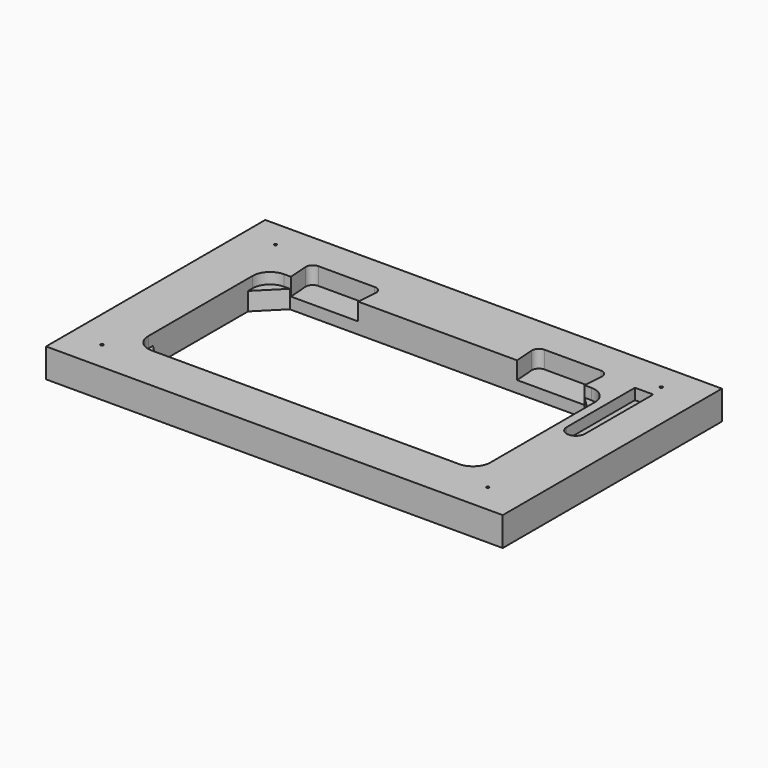
from build123d import *

# Parameters (mm, degrees)
F0_W     = 500
F0_H     = 300
F1_DEPTH = 31.75
F2_R     = 1.5
F3_DEPTH = 31.751
F5_DEPTH = 12
F8_DEPTH = 31.751
F9_DEPTH = 19.05


# Not quite as in the source:
# - a length typed as a fraction of an inch, garbled in the dataset ("3 / 203.2 mm" for 3/8 in), is restored


with BuildPart() as f1:
    # F0 (on Top) → F1 (new body)
    with BuildSketch(Plane.XY):
        Rectangle(F0_W, F0_H)
    extrude(amount=-F1_DEPTH)

    # F2 (on Top) → F3 (cut, through all)
    with BuildSketch(Plane.XY):
        with Locations((-214.6335691214, 119.7834908962)):
            Circle(F2_R)
        with Locations((-214.6335691214, -117.7065091038)):
            Circle(F2_R)
        with Locations((207.7684308786, 119.7834908962)):
            Circle(F2_R)
        with Locations((207.7684308786, -117.7065091038)):
            Circle(F2_R)
        with Locations((630.1704308786, 119.7834908962)):
            Circle(F2_R)
        with Locations((630.1704308786, -117.7065091038)):
            Circle(F2_R)
    extrude(amount=-F3_DEPTH, mode=Mode.SUBTRACT)

    # F4 (on Top) → F5 (cut)
    with BuildSketch(Plane.XY):
        with BuildLine():
            ThreePointArc((-193.759300375, -80.4257169581), (-188.1796845566, -93.8961011397), (-174.709300375, -99.4757169581))
            Line((-174.709300375, -99.4757169581), (161.840699625, -99.4757169581))
            ThreePointArc((161.840699625, -99.4757169581), (175.3110838066, -93.8961011397), (180.890699625, -80.4257169581))
            Line((180.890699625, -80.4257169581), (180.890699625, 62.4492830419))
            ThreePointArc((180.890699625, 62.4492830419), (175.3110838066, 75.9196672235), (161.840699625, 81.4992830419))
            Line((161.840699625, 81.4992830419), (-174.709300375, 81.4992830419))
            ThreePointArc((-174.709300375, 81.4992830419), (-188.1796845566, 75.9196672235), (-193.759300375, 62.4492830419))
            Line((-193.759300375, 62.4492830419), (-193.759300375, -80.4257169581))
        make_face()
        with BuildLine():
            Line((210.890699625, 104.8424765468), (190.890699625, 104.8424765468))
            Line((190.890699625, 104.8424765468), (190.890699625, 11.4992830419))
            ThreePointArc((190.890699625, 11.4992830419), (200.890699625, 1.4992830419), (210.890699625, 11.4992830419))
            Line((210.890699625, 11.4992830419), (210.890699625, 104.8424765468))
        make_face()
    extrude(amount=-F5_DEPTH, mode=Mode.SUBTRACT)

    # F7 (on face) → F8 (cut, through all)
    with BuildSketch(Plane.XY):
        with BuildLine():
            Line((-174.709300375, -93.1257169581), (140.1676505526, -93.1257169581))
            Line((140.1676505526, -93.1257169581), (163.0281784434, -99.438670281))
            ThreePointArc((163.0281784434, -99.438670281), (175.7245746513, -93.4695091312), (180.890699625, -80.4257169581))
            Line((180.890699625, -80.4257169581), (180.890699625, 56.0992830419))
            Line((180.890699625, 56.0992830419), (154.220699625, 81.4992830419))
            Line((154.220699625, 81.4992830419), (-168.359300375, 81.4992830419))
            Line((-168.359300375, 81.4992830419), (-187.409300375, 62.4492830419))
            Line((-187.409300375, 62.4492830419), (-193.759300375, 56.0992830419))
            Line((-193.759300375, 56.0992830419), (-193.759300375, -74.0757169581))
            Line((-193.759300375, -74.0757169581), (-174.709300375, -93.1257169581))
        make_face()
    extrude(amount=-F8_DEPTH, mode=Mode.SUBTRACT)

    # F6 (on Top) → F9 (cut)
    with BuildSketch(Plane.XY):
        with BuildLine():
            ThreePointArc((-161.120300375, 111.4992830419), (-166.7055905698, 109.0628082362), (-168.7191172889, 103.3114965432))
            Line((-168.7191172889, 103.3114965432), (-167.089300375, 81.4992830419))
            Line((-167.089300375, 81.4992830419), (-93.429300375, 81.4992830419))
            Line((-93.429300375, 81.4992830419), (-91.799483461, 103.3114965432))
            ThreePointArc((-91.799483461, 103.3114965432), (-93.8130101802, 109.0628082362), (-99.398300375, 111.4992830419))
            Line((-99.398300375, 111.4992830419), (-161.120300375, 111.4992830419))
        make_face()
        with BuildLine():
            Line((148.251699625, 111.4992830419), (86.529699625, 111.4992830419))
            ThreePointArc((86.529699625, 111.4992830419), (80.9444094302, 109.0628082362), (78.9308827111, 103.3114965432))
            Line((78.9308827111, 103.3114965432), (80.560699625, 81.4992830419))
            Line((80.560699625, 81.4992830419), (154.220699625, 81.4992830419))
            Line((154.220699625, 81.4992830419), (155.850516539, 103.3114965432))
            ThreePointArc((155.850516539, 103.3114965432), (153.8369898198, 109.0628082362), (148.251699625, 111.4992830419))
        make_face()
    extrude(amount=-F9_DEPTH, mode=Mode.SUBTRACT)


solid = f1.part
